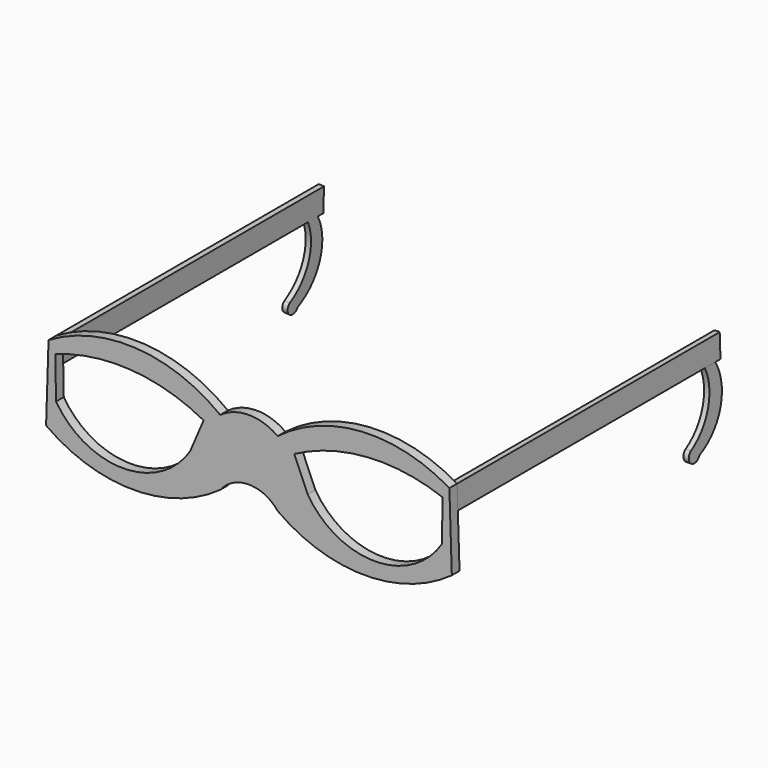
from build123d import *

# Parameters (mm, degrees)
F1_DEPTH  = 2.286
F2_W      = 77.7575820684
F2_H      = 5.6929403374
F3_DEPTH  = 1.27
F4_W      = 77.8131708503
F4_H      = 5.5740863885
F5_DEPTH  = 1.27
F11_DEPTH = 1.27
F12_DEPTH = 1.27


# Not quite as in the source:
# - the program builds the solid bodies; features that only make, move or delete a surface that nothing else refers to are left out


with BuildPart() as f1:
    # F0 (on Front) → F1 (new body)
    with BuildSketch(Plane.XZ):
        with BuildLine():
            ThreePointArc((49.5953476056, 12.2513668612), (28.882888205, 17.3015230489), (8.9030108118, 9.8641477525))
            ThreePointArc((8.9030108118, 9.8641477525), (2.0914725028, 12.0726852219), (-4.7200658062, 9.8641477525))
            ThreePointArc((-4.7200658062, 9.8641477525), (-24.6999431994, 17.3015230489), (-45.4124026, 12.2513668612))
            Line((-45.4124026, 12.2513668612), (-45.9956228733, -5.7643466812))
            ThreePointArc((-45.9956228733, -5.7643466812), (-25.3578443398, -12.4538689532), (-4.7200658062, -5.7643466812))
            ThreePointArc((-4.7200658062, -5.7643466812), (2.0914725028, -2.4552290608), (8.9030108118, -5.7643466812))
            ThreePointArc((8.9030108118, -5.7643466812), (29.5407893454, -12.4538689532), (50.1785678789, -5.7643466812))
            Line((50.1785678789, -5.7643466812), (49.5953476056, 12.2513668612))
        make_face()
        with BuildLine():
            ThreePointArc((-43.8181608915, 9.8152747378), (-25.9821003979, 12.388296488), (-8.655664511, 7.4344985187))
            Line((-8.655664511, 7.4344985187), (-11.8352537975, 0))
            ThreePointArc((-11.8352537975, 0), (-27.7331932448, -8.7587656644), (-43.6311326921, 0))
            Line((-43.6311326921, 0), (-43.8181608915, 9.8152747378))
        make_face(mode=Mode.SUBTRACT)
        with BuildLine():
            Line((48.0011058971, 9.8152747378), (47.8140776977, 0))
            ThreePointArc((47.8140776977, 0), (31.9161382504, -8.7587656644), (16.0181988031, 0))
            Line((16.0181988031, 0), (12.8386095166, 7.4344985187))
            ThreePointArc((12.8386095166, 7.4344985187), (30.1650454035, 12.388296488), (48.0011058971, 9.8152747378))
        make_face(mode=Mode.SUBTRACT)
    extrude(amount=F1_DEPTH)

    # F2 (on face) → F3 (join)
    with BuildSketch(Plane(origin=(-45.7610567543, 0, 1.4814165402), x_dir=(0, -1, 0), z_dir=(-0.9994764103, 0, 0.0323559155))):
        with Locations((-38.8787910342, 7.9291221415)):
            Rectangle(F2_W, F2_H)
    extrude(amount=-F3_DEPTH)

    # F4 (on face) → F5 (join)
    with BuildSketch(Plane(origin=(49.9396226128, 0, 1.6166886911), x_dir=(0, 1, 0), z_dir=(0.9994764103, 0, 0.0323559155))):
        with Locations((38.9065854251, 7.8532061008)):
            Rectangle(F4_W, F4_H)
    extrude(amount=-F5_DEPTH)

    # F10 (on face) → F11 (join)
    with BuildSketch(Plane(origin=(-45.7610567543, 0, 1.4814165402), x_dir=(0, -1, 0), z_dir=(-0.9994764103, 0, 0.0323559155))):
        with BuildLine():
            ThreePointArc((-68.4109553695, -10.0245960057), (-73.7805543262, -3.4143727695), (-73.2076540589, 5.0826519728))
            Line((-73.2076540589, 5.0826519728), (-76.1324688792, 5.0826519728))
            ThreePointArc((-76.1324688792, 5.0826519728), (-77.1679356937, -4.5445995463), (-70.867806673, -11.8974586949))
            ThreePointArc((-70.867806673, -11.8974586949), (-68.4698563349, -12.4952285851), (-68.4109553695, -10.0245960057))
        make_face()
    extrude(amount=-F11_DEPTH)


with BuildPart() as f12:
    # F9 (on face) → F12 (new body)
    with BuildSketch(Plane(origin=(49.9396226128, 0, 1.6166886911), x_dir=(0, 1, 0), z_dir=(0.9994764103, 0, 0.0323559155))):
        with BuildLine():
            ThreePointArc((68.4109553695, -10.1599385962), (68.3834154508, -12.7439657132), (70.867806673, -12.0328012854))
            ThreePointArc((70.867806673, -12.0328012854), (77.4354700769, -4.7034982276), (76.2494653463, 5.0661629066))
            Line((76.2494653463, 5.0661629066), (73.2076540589, 5.0661629066))
            ThreePointArc((73.2076540589, 5.0661629066), (73.7912313756, -3.4862881047), (68.4109553695, -10.1599385962))
        make_face()
    extrude(amount=-F12_DEPTH)


solid = Compound([f1.part, f12.part])
